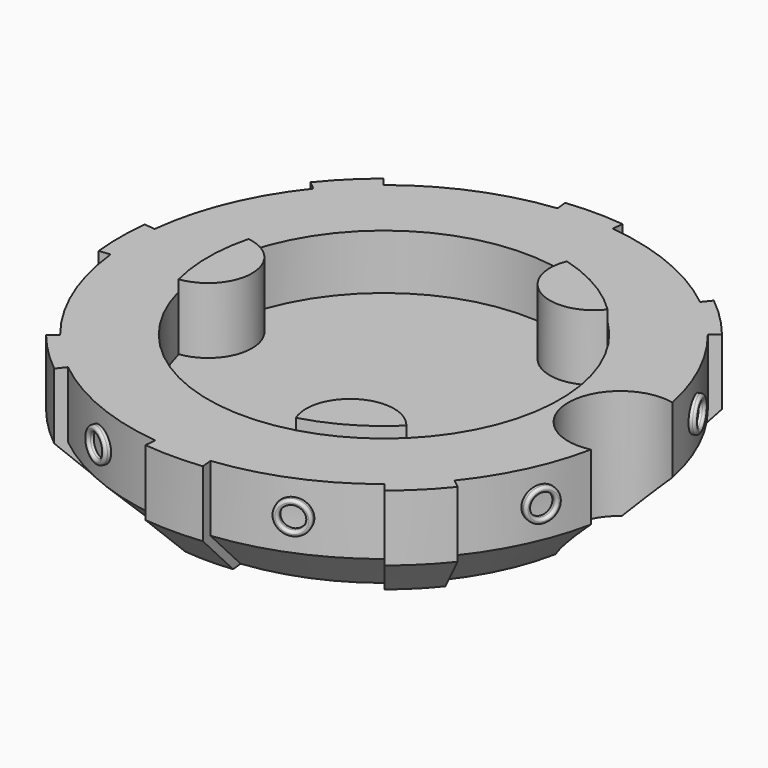
from build123d import *

# Parameters (mm, degrees)
F3_ANGLE_BACK  = 6.25
F3_ANGLE       = 12.5
F7_R           = 4.7625
F7_R_2         = 3.175
F8_DEPTH       = 3.175
F9_R           = 0.79374
F10_COUNT      = 8
F11_R          = 50.8
F12_DEPTH      = 3.175
F14_DEPTH      = 15.875
F14_DEPTH_BACK = 3.175
F16_R          = 15.08125
F17_DEPTH      = 31.75


# Not quite as in the source:
# - a fillet or chamfer is up to 0.001 mm smaller than in the source, because OpenCascade refuses the exact size


with BuildPart() as f1:
    # F0 (on Front) → F1 (revolve)
    with BuildSketch(Plane.XZ):
        Polygon((-50.8, 19.05), (-73.025, 19.05), (-73.025, 0), (-60.325, -12.7), (-50.8, -12.7), align=None)
    revolve(axis=Axis((0, 0, 4.5524518511), (0, 0, -1)))

    # F2 (on Front) → F3 (revolve)
    with BuildSketch(Plane.XZ, mode=Mode.PRIVATE) as f3_sk:
        Polygon((-73.025, 0), (-73.025, 19.05), (-76.2, 19.05), (-76.2, 0), (-63.5, -12.7), (-60.325, -12.7), align=None)
    revolve(f3_sk.sketch.rotate(Axis((0, 0, 4.5524518511), (0, 0, -1)), -F3_ANGLE_BACK), axis=Axis((0, 0, 4.5524518511), (0, 0, -1)), revolution_arc=F3_ANGLE)

    # F7 (on face) → F8 (join)
    with BuildSketch(Plane(origin=(-68.9329616195, -28.5529675973, 0), x_dir=(0.3826834324, -0.9238795325, 0), z_dir=(-0.9238795325, -0.3826834324, 0))):
        with Locations((0, 9.525)):
            Circle(F7_R)
        with Locations((0, 9.525)):
            Circle(F7_R_2, mode=Mode.SUBTRACT)
    extrude(amount=-F8_DEPTH)

    # F9 (radius 0.79375 in the source; OpenCascade refuses exactly that, so slightly less here)
    f9_edges = [f1.edges().sort_by_distance(p)[0] for p in [
        (-70.755491, -24.152991, 9.525),
        (-70.147982, -25.61965, 9.525),
    ]]
    fillet(f9_edges, radius=F9_R)


with BuildPart() as f10_1:
    # F10: instance of F1
    add(f1.part.rotate(Axis((0, 0, 4.5524518511), (0, 0, -1)), 1 * 360 / F10_COUNT))


with BuildPart() as f10_2:
    # F10: instance of F1
    add(f1.part.rotate(Axis((0, 0, 4.5524518511), (0, 0, -1)), 2 * 360 / F10_COUNT))


with BuildPart() as f10_3:
    # F10: instance of F1
    add(f1.part.rotate(Axis((0, 0, 4.5524518511), (0, 0, -1)), 3 * 360 / F10_COUNT))


with BuildPart() as f10_4:
    # F10: instance of F1
    add(f1.part.rotate(Axis((0, 0, 4.5524518511), (0, 0, -1)), 4 * 360 / F10_COUNT))


with BuildPart() as f10_5:
    # F10: instance of F1
    add(f1.part.rotate(Axis((0, 0, 4.5524518511), (0, 0, -1)), 5 * 360 / F10_COUNT))


with BuildPart() as f10_6:
    # F10: instance of F1
    add(f1.part.rotate(Axis((0, 0, 4.5524518511), (0, 0, -1)), 6 * 360 / F10_COUNT))


with BuildPart() as f10_7:
    # F10: instance of F1
    add(f1.part.rotate(Axis((0, 0, 4.5524518511), (0, 0, -1)), 7 * 360 / F10_COUNT))


with BuildPart() as f1_1:
    add(f1.part)

    add(f10_1.part)  # F12 merges F10_1

    add(f10_2.part)  # F12 merges F10_2

    add(f10_3.part)  # F12 merges F10_3

    add(f10_4.part)  # F12 merges F10_4

    add(f10_5.part)  # F12 merges F10_5

    add(f10_6.part)  # F12 merges F10_6

    add(f10_7.part)  # F12 merges F10_7
    # F11 (on Top) → F12 (join)
    with BuildSketch(Plane.XY):
        Circle(F11_R)
    extrude(amount=F12_DEPTH)

    # F13 (on face) → F14 (join, two sides)
    with BuildSketch(Plane.XY.offset(19.05)) as f14_sk:
        with BuildLine():
            ThreePointArc((-49.2125, -12.6003906189), (-38.1, 0), (-49.2125, 12.6003906189))
            ThreePointArc((-49.2125, 12.6003906189), (-50.8, 0), (-49.2125, -12.6003906189))
        make_face()
        with BuildLine():
            ThreePointArc((35.5185083736, 36.3190798743), (25.4, 43.9940905122), (13.6939916264, 48.9194704932))
            ThreePointArc((13.6939916264, 48.9194704932), (19.05, 32.9955678842), (35.5185083736, 36.3190798743))
        make_face()
        with BuildLine():
            ThreePointArc((35.5185083736, -36.3190798743), (19.05, -32.9955678842), (13.6939916264, -48.9194704932))
            ThreePointArc((13.6939916264, -48.9194704932), (25.4, -43.9940905122), (35.5185083736, -36.3190798743))
        make_face()
    extrude(amount=-F14_DEPTH)
    extrude(f14_sk.sketch, amount=F14_DEPTH_BACK)

    # F15: union 

    # F16 (on face) → F17 (cut)
    with BuildSketch(Plane.XY.offset(19.05)):
        with Locations((68.2625, 0)):
            Circle(F16_R)
    extrude(amount=-F17_DEPTH, mode=Mode.SUBTRACT)


solid = f1_1.part
